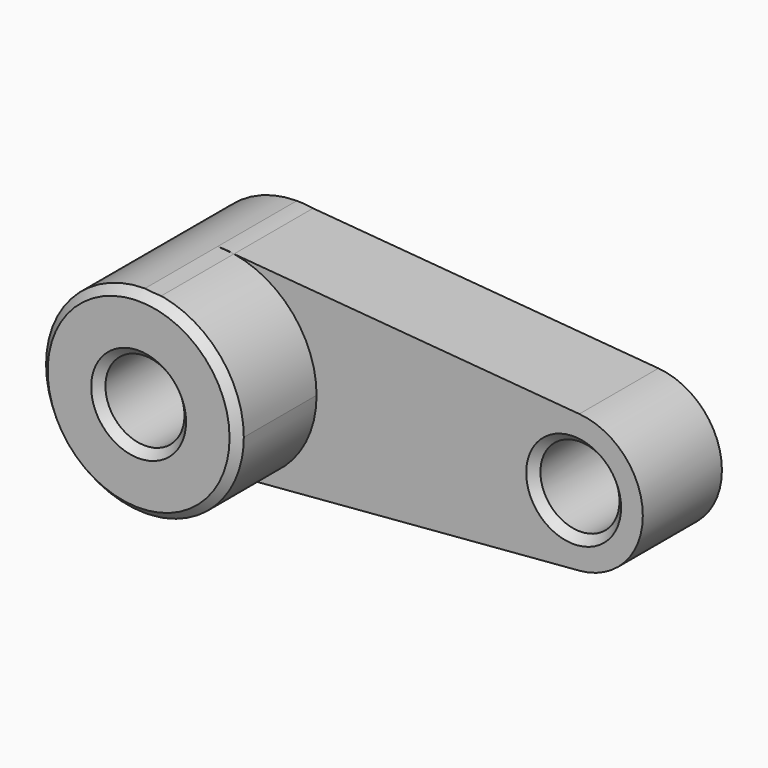
from build123d import *

# Parameters (mm, degrees)
F0_R        = 10
F1_DEPTH    = 25
F2_DEPTH    = 50
F3_T6_ANGLE = 203.6133668192
F3_T8_ANGLE = 179.9906971182


# Not quite as in the source:
# - a fillet or chamfer that OpenCascade refuses, or shapes differently, is made with other operations: its cross-section is extruded or revolved along the edge and cut away or added


with BuildPart() as f1:
    # F0 (on Front) → F1 (new body)
    with BuildSketch(Plane.XZ):
        with BuildLine():
            Line((4.1054428346, 24.6606029758), (0, 25))
            ThreePointArc((0, 25), (-25, 0), (0, -25))
            Line((0, -25), (4.1054428346, -24.6606029758))
            ThreePointArc((4.1054428346, -24.6606029758), (19.0740146648, -16.1611251022), (25, 0))
            ThreePointArc((25, 0), (19.0740146648, 16.1611251022), (4.1054428346, 24.6606029758))
        make_face()
        Circle(F0_R, mode=Mode.SUBTRACT)
        with BuildLine():
            ThreePointArc((4.1054428346, 24.6606029758), (2.0597239626, 24.9150062653), (0, 25))
            Line((0, 25), (4.1054428346, 24.6606029758))
        make_face()
        with BuildLine():
            Line((4.1054428346, -24.6606029758), (0, -25))
            ThreePointArc((0, -25), (2.0597239626, -24.9150062653), (4.1054428346, -24.6606029758))
        make_face()
        with BuildLine():
            Line((91.4418067738, 17.4405043857), (4.1054428346, 24.6606029758))
            ThreePointArc((4.1054428346, 24.6606029758), (19.0740146648, 16.1611251022), (25, 0))
            ThreePointArc((25, 0), (19.0740146648, -16.1611251022), (4.1054428346, -24.6606029758))
            Line((4.1054428346, -24.6606029758), (91.4418067738, -17.4405043857))
            ThreePointArc((91.4418067738, -17.4405043857), (72.5, 0), (91.4418067738, 17.4405043857))
        make_face()
        with BuildLine():
            ThreePointArc((107.5, 0), (102.8740362463, 11.8536572723), (91.4418067738, 17.4405043857))
            ThreePointArc((91.4418067738, 17.4405043857), (72.5, 0), (91.4418067738, -17.4405043857))
            ThreePointArc((91.4418067738, -17.4405043857), (102.8740362463, -11.8536572723), (107.5, 0))
        make_face()
        with Locations((90, 0)):
            Circle(F0_R, mode=Mode.SUBTRACT)
    extrude(amount=F1_DEPTH)

    # F0 (on Front) → F2 (join)
    with BuildSketch(Plane.XZ):
        with BuildLine():
            Line((4.1054428346, 24.6606029758), (0, 25))
            ThreePointArc((0, 25), (-25, 0), (0, -25))
            Line((0, -25), (4.1054428346, -24.6606029758))
            ThreePointArc((4.1054428346, -24.6606029758), (19.0740146648, -16.1611251022), (25, 0))
            ThreePointArc((25, 0), (19.0740146648, 16.1611251022), (4.1054428346, 24.6606029758))
        make_face()
        Circle(F0_R, mode=Mode.SUBTRACT)
    extrude(amount=F2_DEPTH)

    # F3: chamfer of 2 on 8 edges, made by hand

    # F3_s1 → F3_t2 (revolve, cut)
    with BuildSketch(Plane.XY):
        with BuildLine():
            Line((9.9434314575, -2.0565685425), (12.0565685425, 0.0565685425))
            Line((12.0565685425, 0.0565685425), (12.0565685425, 0.0965685425))
            ThreePointArc((12.0565685425, 0.0965685425), (11.0282842712, 0.04), (10, 0.04))
            Line((10, 0.04), (9.96, 0))
            ThreePointArc((9.96, 0), (9.96, -1.0282842712), (9.9034314575, -2.0565685425))
            Line((9.9034314575, -2.0565685425), (9.9434314575, -2.0565685425))
        make_face()
    revolve(axis=Axis((0, 0, 0), (0, -1, 0)), mode=Mode.SUBTRACT)

    # F3_s3 → F3_t4 (revolve, cut)
    with BuildSketch(Plane.XY):
        with BuildLine():
            Line((12.0565685425, -50.0565685425), (9.9434314575, -47.9434314575))
            Line((9.9434314575, -47.9434314575), (9.9034314575, -47.9434314575))
            ThreePointArc((9.9034314575, -47.9434314575), (9.96, -48.9717157288), (9.96, -50))
            Line((9.96, -50), (10, -50.04))
            ThreePointArc((10, -50.04), (11.0282842712, -50.04), (12.0565685425, -50.0965685425))
            Line((12.0565685425, -50.0965685425), (12.0565685425, -50.0565685425))
        make_face()
    revolve(axis=Axis((0, -50, 0), (0, -1, 0)), mode=Mode.SUBTRACT)

    # F3_s5 → F3_t6 (revolve, cut)
    with BuildSketch(Plane(origin=(0, 0, 0), x_dir=(0, 1, 0), z_dir=(0.9788435281, 0, -0.2046102329))):
        with BuildLine():
            Line((-47.9434314575, 25.0565685425), (-50.0565685425, 22.9434314575))
            Line((-50.0565685425, 22.9434314575), (-50.0965685425, 22.9434314575))
            ThreePointArc((-50.0965685425, 22.9434314575), (-50.04, 23.9717157288), (-50.04, 25))
            Line((-50.04, 25), (-50, 25.04))
            ThreePointArc((-50, 25.04), (-48.9717157288, 25.04), (-47.9434314575, 25.0965685425))
            Line((-47.9434314575, 25.0965685425), (-47.9434314575, 25.0565685425))
        make_face()
    revolve(axis=Axis((0, -50, 0), (0, -1, 0)), revolution_arc=F3_T6_ANGLE, mode=Mode.SUBTRACT)

    # F3_s7 → F3_t8 (revolve, cut)
    with BuildSketch(Plane(origin=(0, 0, 0), x_dir=(0, 1, 0), z_dir=(-0.9999999967, 0, 8.1183e-05))):
        with BuildLine():
            Line((-47.9434314575, -25.0565685425), (-50.0565685425, -22.9434314575))
            Line((-50.0565685425, -22.9434314575), (-50.0965685425, -22.9434314575))
            ThreePointArc((-50.0965685425, -22.9434314575), (-50.04, -23.9717157288), (-50.04, -25))
            Line((-50.04, -25), (-50, -25.04))
            ThreePointArc((-50, -25.04), (-48.9717157288, -25.04), (-47.9434314575, -25.0965685425))
            Line((-47.9434314575, -25.0965685425), (-47.9434314575, -25.0565685425))
        make_face()
    revolve(axis=Axis((0, -50, 0), (0, 1, 0)), revolution_arc=F3_T8_ANGLE, mode=Mode.SUBTRACT)

    # F3_s9 → F3_t10 (revolve, cut)
    with BuildSketch(Plane.XY):
        with BuildLine():
            Line((99.9434314575, -2.0565685425), (102.0565685425, 0.0565685425))
            Line((102.0565685425, 0.0565685425), (102.0565685425, 0.0965685425))
            ThreePointArc((102.0565685425, 0.0965685425), (101.0282842712, 0.04), (100, 0.04))
            Line((100, 0.04), (99.96, 0))
            ThreePointArc((99.96, 0), (99.96, -1.0282842712), (99.9034314575, -2.0565685425))
            Line((99.9034314575, -2.0565685425), (99.9434314575, -2.0565685425))
        make_face()
    revolve(axis=Axis((90, 0, 0), (0, -1, 0)), mode=Mode.SUBTRACT)

    # F3_s11 → F3_t12 (revolve, cut)
    with BuildSketch(Plane.XY):
        with BuildLine():
            Line((102.0565685425, -25.0565685425), (99.9434314575, -22.9434314575))
            Line((99.9434314575, -22.9434314575), (99.9034314575, -22.9434314575))
            ThreePointArc((99.9034314575, -22.9434314575), (99.96, -23.9717157288), (99.96, -25))
            Line((99.96, -25), (100, -25.04))
            ThreePointArc((100, -25.04), (101.0282842712, -25.04), (102.0565685425, -25.0965685425))
            Line((102.0565685425, -25.0965685425), (102.0565685425, -25.0565685425))
        make_face()
    revolve(axis=Axis((90, -25, 0), (0, -1, 0)), mode=Mode.SUBTRACT)


solid = f1.part
